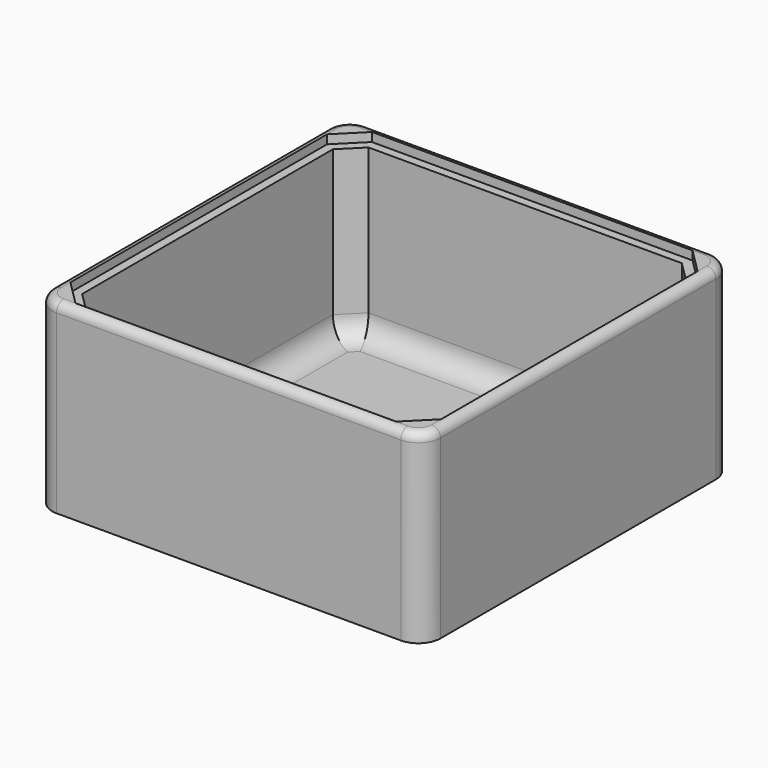
from build123d import *

# Parameters (mm, degrees)
F1_DEPTH = 40
F2_DEPTH = 38
F3_DEPTH = 2
F4_R     = 1.99999
F5_R     = 5


# Not quite as in the source:
# - a fillet or chamfer is up to 0.001 mm smaller than in the source, because OpenCascade refuses the exact size


with BuildPart() as f1:
    # F0 (on Top) → F1 (new body)
    with BuildSketch(Plane.XY):
        with BuildLine():
            Line((-39, -44), (39, -44))
            ThreePointArc((39, -44), (42.5355339059, -42.5355339059), (44, -39))
            Line((44, -39), (44, 39))
            ThreePointArc((44, 39), (42.5355339059, 42.5355339059), (39, 44))
            Line((39, 44), (-39, 44))
            ThreePointArc((-39, 44), (-42.5355339059, 42.5355339059), (-44, 39))
            Line((-44, 39), (-44, -39))
            ThreePointArc((-44, -39), (-42.5355339059, -42.5355339059), (-39, -44))
        make_face()
        Polygon((42, -36.3431457505), (42, -42), (36.3431457505, -42), (-36.3431457505, -42), (-42, -42), (-42, -36.3431457505), (-42, 36.3431457505), (-42, 42), (-36.3431457505, 42), (36.3431457505, 42), (42, 42), (42, 36.3431457505), align=None, mode=Mode.SUBTRACT)
        Polygon((-35.5147186258, -40), (35.5147186258, -40), (40, -35.5147186258), (40, 35.5147186258), (35.5147186258, 40), (-35.5147186258, 40), (-40, 35.5147186258), (-40, -35.5147186258), align=None)
        Polygon((40, 35.5147186258), (40, 38.3431457505), (38.3431457505, 40), (35.5147186258, 40), align=None)
        Polygon((40, 38.3431457505), (42, 36.3431457505), (42, 42), (36.3431457505, 42), (38.3431457505, 40), (40, 40), align=None)
        Polygon((38.3431457505, 40), (40, 38.3431457505), (40, 40), align=None)
        Polygon((40, -38.3431457505), (42, -36.3431457505), (42, 36.3431457505), (40, 38.3431457505), (40, 35.5147186258), (40, -35.5147186258), align=None)
        Polygon((38.3431457505, 40), (36.3431457505, 42), (-36.3431457505, 42), (-38.3431457505, 40), (-35.5147186258, 40), (35.5147186258, 40), align=None)
        Polygon((-38.3431457505, 40), (-40, 38.3431457505), (-40, 35.5147186258), (-35.5147186258, 40), align=None)
        Polygon((-40, 40), (-40, 38.3431457505), (-38.3431457505, 40), align=None)
        Polygon((-42, 42), (-42, 36.3431457505), (-40, 38.3431457505), (-40, 40), (-38.3431457505, 40), (-36.3431457505, 42), align=None)
        Polygon((-42, 36.3431457505), (-42, -36.3431457505), (-40, -38.3431457505), (-40, -35.5147186258), (-40, 35.5147186258), (-40, 38.3431457505), align=None)
        Polygon((-40, -38.3431457505), (-38.3431457505, -40), (-35.5147186258, -40), (-40, -35.5147186258), align=None)
        Polygon((-40, -40), (-38.3431457505, -40), (-40, -38.3431457505), align=None)
        Polygon((-42, -42), (-36.3431457505, -42), (-38.3431457505, -40), (-40, -40), (-40, -38.3431457505), (-42, -36.3431457505), align=None)
        Polygon((-36.3431457505, -42), (36.3431457505, -42), (38.3431457505, -40), (35.5147186258, -40), (-35.5147186258, -40), (-38.3431457505, -40), align=None)
        Polygon((35.5147186258, -40), (38.3431457505, -40), (40, -38.3431457505), (40, -35.5147186258), align=None)
        Polygon((40, -38.3431457505), (38.3431457505, -40), (40, -40), align=None)
        Polygon((36.3431457505, -42), (42, -42), (42, -36.3431457505), (40, -38.3431457505), (40, -40), (38.3431457505, -40), align=None)
    extrude(amount=-F1_DEPTH)

    # F0 (on Top) → F2 (cut)
    with BuildSketch(Plane.XY):
        Polygon((-35.5147186258, -40), (35.5147186258, -40), (40, -35.5147186258), (40, 35.5147186258), (35.5147186258, 40), (-35.5147186258, 40), (-40, 35.5147186258), (-40, -35.5147186258), align=None)
    extrude(amount=-F2_DEPTH, mode=Mode.SUBTRACT)

    # F0 (on Top) → F3 (join)
    with BuildSketch(Plane.XY):
        with BuildLine():
            Line((-39, -44), (39, -44))
            ThreePointArc((39, -44), (42.5355339059, -42.5355339059), (44, -39))
            Line((44, -39), (44, 39))
            ThreePointArc((44, 39), (42.5355339059, 42.5355339059), (39, 44))
            Line((39, 44), (-39, 44))
            ThreePointArc((-39, 44), (-42.5355339059, 42.5355339059), (-44, 39))
            Line((-44, 39), (-44, -39))
            ThreePointArc((-44, -39), (-42.5355339059, -42.5355339059), (-39, -44))
        make_face()
        Polygon((42, -36.3431457505), (42, -42), (36.3431457505, -42), (-36.3431457505, -42), (-42, -42), (-42, -36.3431457505), (-42, 36.3431457505), (-42, 42), (-36.3431457505, 42), (36.3431457505, 42), (42, 42), (42, 36.3431457505), align=None, mode=Mode.SUBTRACT)
        Polygon((-42, 42), (-42, 36.3431457505), (-40, 38.3431457505), (-40, 40), (-38.3431457505, 40), (-36.3431457505, 42), align=None)
        Polygon((-40, 40), (-40, 38.3431457505), (-38.3431457505, 40), align=None)
        Polygon((40, 38.3431457505), (42, 36.3431457505), (42, 42), (36.3431457505, 42), (38.3431457505, 40), (40, 40), align=None)
        Polygon((38.3431457505, 40), (40, 38.3431457505), (40, 40), align=None)
        Polygon((36.3431457505, -42), (42, -42), (42, -36.3431457505), (40, -38.3431457505), (40, -40), (38.3431457505, -40), align=None)
        Polygon((40, -38.3431457505), (38.3431457505, -40), (40, -40), align=None)
        Polygon((-42, -42), (-36.3431457505, -42), (-38.3431457505, -40), (-40, -40), (-40, -38.3431457505), (-42, -36.3431457505), align=None)
        Polygon((-40, -40), (-38.3431457505, -40), (-40, -38.3431457505), align=None)
    extrude(amount=F3_DEPTH)

    # F4 (radius 2 in the source; OpenCascade refuses exactly that, so slightly less here)
    f4_edges = [f1.edges().sort_by_distance(p)[0] for p in [
        (-42.535534, -42.535534, 2),
    ]]
    fillet(f4_edges, radius=F4_R)

    # F5
    f5_edges = [f1.edges().sort_by_distance(p)[0] for p in [
        (0, 40, -38),
        (-40, 0, -38),
        (-37.757359, 37.757359, -38),
        (-37.757359, -37.757359, -38),
        (0, -40, -38),
        (37.757359, -37.757359, -38),
        (40, 0, -38),
        (37.757359, 37.757359, -38),
    ]]
    fillet(f5_edges, radius=F5_R)


solid = f1.part
